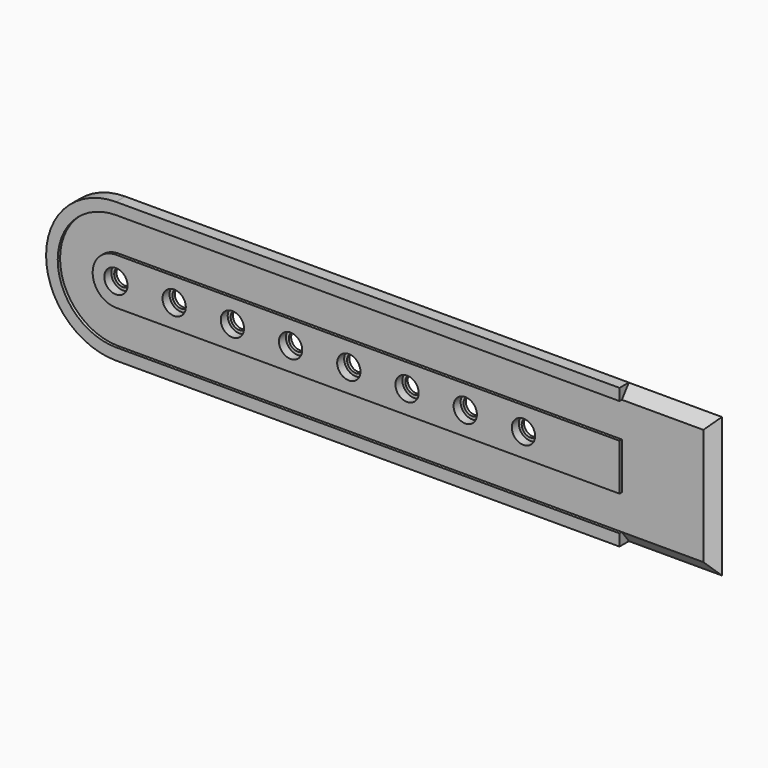
from build123d import *

# Parameters (mm, degrees)
F1_DEPTH     = 1.5875
F2_DEPTH     = 1.18872
F0_R         = 1.5875
F3_DEPTH     = 1.5875
F0_R_2       = 1.190625
F4_DEPTH     = 0.39624
F5_DEPTH     = 1.18872
F6_T1_DEPTH  = 27.2432951274
F6_T6_DEPTH  = 16.7966475637
F6_T11_DEPTH = 16.7966475637


# Not quite as in the source:
# - a fillet or chamfer that OpenCascade refuses, or shapes differently, is made with other operations: its cross-section is extruded or revolved along the edge and cut away or added


with BuildPart() as f1:
    # F0 (on Front) → F1 (new body)
    with BuildSketch(Plane.XZ):
        with BuildLine():
            Line((-81.3593362805, 0), (-12.7, 0))
            Line((-12.7, 0), (-12.7, 1.5875))
            Line((-12.7, 1.5875), (-81.3593362805, 1.5875))
            ThreePointArc((-81.3593362805, 1.5875), (-89.2968362805, 9.525), (-81.3593362805, 17.4625))
            Line((-81.3593362805, 17.4625), (-12.7, 17.4625))
            Line((-12.7, 17.4625), (-12.7, 19.05))
            Line((-12.7, 19.05), (-81.3593362805, 19.05))
            ThreePointArc((-81.3593362805, 19.05), (-90.8843362805, 9.525), (-81.3593362805, 0))
        make_face()
    extrude(amount=F1_DEPTH)

    # F0 (on Front) → F2 (join)
    with BuildSketch(Plane.XZ):
        with BuildLine():
            Line((-81.3593362805, 1.5875), (-12.7, 1.5875))
            Line((-12.7, 1.5875), (-1.5875, 1.5875))
            Line((-1.5875, 1.5875), (-1.5875, 17.4625))
            Line((-1.5875, 17.4625), (-12.7, 17.4625))
            Line((-12.7, 17.4625), (-81.3593362805, 17.4625))
            ThreePointArc((-81.3593362805, 17.4625), (-89.2968362805, 9.525), (-81.3593362805, 1.5875))
        make_face()
        with BuildLine():
            ThreePointArc((-81.3593362805, 6.35), (-84.5343362805, 9.525), (-81.3593362805, 12.7))
            Line((-81.3593362805, 12.7), (-12.7, 12.7))
            Line((-12.7, 12.7), (-12.7, 6.35))
            Line((-12.7, 6.35), (-81.3593362805, 6.35))
        make_face(mode=Mode.SUBTRACT)
    extrude(amount=F2_DEPTH)

    # F0 (on Front) → F3 (join)
    with BuildSketch(Plane.XZ):
        with BuildLine():
            Line((-12.7, 12.7), (-81.3593362805, 12.7))
            ThreePointArc((-81.3593362805, 12.7), (-84.5343362805, 9.525), (-81.3593362805, 6.35))
            Line((-81.3593362805, 6.35), (-12.7, 6.35))
            Line((-12.7, 6.35), (-12.7, 12.7))
        make_face()
        with Locations((-81.3593362805, 9.525)):
            Circle(F0_R, mode=Mode.SUBTRACT)
        with Locations((-73.4218362805, 9.525)):
            Circle(F0_R, mode=Mode.SUBTRACT)
        with Locations((-65.4843362805, 9.525)):
            Circle(F0_R, mode=Mode.SUBTRACT)
        with Locations((-57.5468362805, 9.525)):
            Circle(F0_R, mode=Mode.SUBTRACT)
        with Locations((-49.6093362805, 9.525)):
            Circle(F0_R, mode=Mode.SUBTRACT)
        with Locations((-41.6718362805, 9.525)):
            Circle(F0_R, mode=Mode.SUBTRACT)
        with Locations((-33.7343362805, 9.525)):
            Circle(F0_R, mode=Mode.SUBTRACT)
        with Locations((-25.7968362805, 9.525)):
            Circle(F0_R, mode=Mode.SUBTRACT)
    extrude(amount=F3_DEPTH)

    # F0 (on Front) → F4 (join)
    with BuildSketch(Plane.XZ):
        with Locations((-81.3593362805, 9.525)):
            Circle(F0_R)
        with Locations((-81.3593362805, 9.525)):
            Circle(F0_R_2, mode=Mode.SUBTRACT)
        with Locations((-73.4218362805, 9.525)):
            Circle(F0_R)
        with Locations((-73.4218362805, 9.525)):
            Circle(F0_R_2, mode=Mode.SUBTRACT)
        with Locations((-65.4843362805, 9.525)):
            Circle(F0_R)
        with Locations((-65.4843362805, 9.525)):
            Circle(F0_R_2, mode=Mode.SUBTRACT)
        with Locations((-57.5468362805, 9.525)):
            Circle(F0_R)
        with Locations((-57.5468362805, 9.525)):
            Circle(F0_R_2, mode=Mode.SUBTRACT)
        with Locations((-49.6093362805, 9.525)):
            Circle(F0_R)
        with Locations((-49.6093362805, 9.525)):
            Circle(F0_R_2, mode=Mode.SUBTRACT)
        with Locations((-41.6718362805, 9.525)):
            Circle(F0_R)
        with Locations((-41.6718362805, 9.525)):
            Circle(F0_R_2, mode=Mode.SUBTRACT)
        with Locations((-33.7343362805, 9.525)):
            Circle(F0_R)
        with Locations((-33.7343362805, 9.525)):
            Circle(F0_R_2, mode=Mode.SUBTRACT)
        with Locations((-25.7968362805, 9.525)):
            Circle(F0_R)
        with Locations((-25.7968362805, 9.525)):
            Circle(F0_R_2, mode=Mode.SUBTRACT)
    extrude(amount=F4_DEPTH)

    # F0 (on Front) → F5 (join)
    with BuildSketch(Plane.XZ):
        Polygon((-12.7, 0), (0, 0), (0, 19.05), (-12.7, 19.05), (-12.7, 17.4625), (-1.5875, 17.4625), (-1.5875, 1.5875), (-12.7, 1.5875), align=None)
    extrude(amount=F5_DEPTH)

    # F6: chamfer of 1.5875 x 1.1962670545 on 3 edges, made by hand

    # F6_s2 → F6_t1 (cut)
    with BuildSketch(Plane.XY.offset(-4.0966475637)):
        Polygon((-1.5875, -1.18872), (0, 0.0075470545), (0, -1.18872), align=None)
    extrude(amount=F6_T1_DEPTH, mode=Mode.SUBTRACT)


with BuildPart() as f6_tool4:
    # F6_s5 → F6_t6 (new body)
    with BuildSketch(Plane.YZ.offset(4.0966475637)):
        Polygon((-1.18872, 17.4625), (0.0075470545, 19.05), (-1.18872, 19.05), align=None)
    extrude(amount=-F6_T6_DEPTH)

    split(bisect_by=Plane.XY.offset(17.4625), keep=Keep.TOP)


with BuildPart() as f1_1:
    add(f1.part)

    # F6_t3: cut F6_tool4
    add(f6_tool4.part, mode=Mode.SUBTRACT)


with BuildPart() as f6_tool9:
    # F6_s10 → F6_t11 (new body)
    with BuildSketch(Plane.YZ.offset(-12.7)):
        Polygon((-1.18872, 1.5875), (0.0075470545, 0), (-1.18872, 0), align=None)
    extrude(amount=F6_T11_DEPTH)

    split(bisect_by=Plane.XY.offset(1.5875), keep=Keep.BOTTOM)


with BuildPart() as f1_2:
    add(f1_1.part)

    # F6_t8: cut F6_tool9
    add(f6_tool9.part, mode=Mode.SUBTRACT)


solid = f1_2.part
